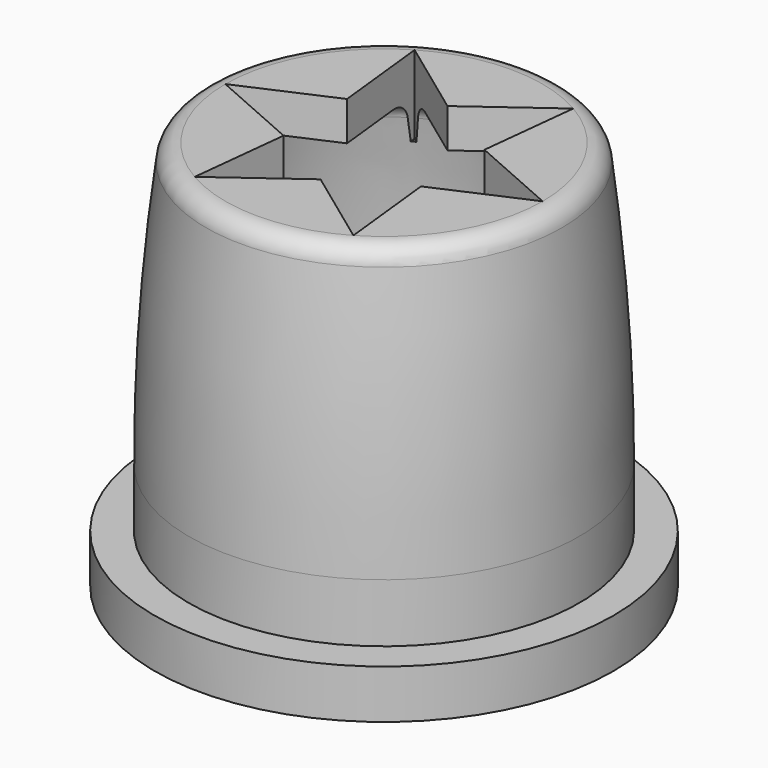
from build123d import *

# Parameters (mm, degrees)
F3_DEPTH    = 4
F4_S6_R     = 8.85
F4_T7_DEPTH = 16


# Not quite as in the source:
# - a fillet or chamfer that OpenCascade refuses, or shapes differently, is made with other operations: its cross-section is extruded or revolved along the edge and cut away or added


with BuildPart() as f1:
    # F0 (on Front) → F1 (revolve)
    with BuildSketch(Plane.XZ):
        with BuildLine():
            Line((-11.75, 2.5), (-11.75, 0))
            Line((-11.75, 0), (-10.45, 0))
            Line((-10.45, 0), (-10.45, 1.2))
            Line((-10.45, 1.2), (-8.85, 1.2))
            Line((-8.85, 1.2), (-8.85, 4.2))
            ThreePointArc((-8.85, 4.2), (-8.5510140246, 10.7185269337), (-7.6565668329, 17.1823145401))
            ThreePointArc((-7.6565668329, 17.1823145401), (-7.3127346822, 17.7688675244), (-6.6733265732, 18))
            Line((-6.6733265732, 18), (0, 18))
            Line((0, 18), (0, 20))
            Line((0, 20), (-8.1253765053, 20))
            ThreePointArc((-8.1253765053, 20), (-8.7852885229, 19.7513428838), (-9.117016902, 19.1290322581))
            ThreePointArc((-9.117016902, 19.1290322581), (-9.7790230738, 12.3288025935), (-10, 5.5))
            Line((-10, 5.5), (-10, 2.5))
            Line((-10, 2.5), (-11.75, 2.5))
        make_face()
    revolve(axis=Axis((0, 0, 19), (0, 0, -1)))

    # F2 (on face) → F3 (cut)
    with BuildSketch(Plane.XY.offset(20)):
        Polygon((4.0626882527, 7.0367824689), (0, 4.0626882527), (-4.0626882527, 7.0367824689), (-3.5183912345, 2.0313441263), (-8.1253765053, 0), (-3.5183912345, -2.0313441263), (-4.0626882527, -7.0367824689), (0, -4.0626882527), (4.0626882527, -7.0367824689), (3.5183912345, -2.0313441263), (8.1253765053, 0), (3.5183912345, 2.0313441263), align=None)
    extrude(amount=-F3_DEPTH, mode=Mode.SUBTRACT)

    # F4: chamfer of 2 on 1 edges, made by hand


with BuildPart() as f4_tool2:
    # F4_s3 → F4_t4 (revolve)
    with BuildSketch(Plane.XZ):
        Polygon((-10.45, -0.8), (-8.45, 1.2), (-10.45, 1.2), align=None)
    revolve(axis=Axis((0, 0, 1.2), (0, 0, -1)))

    split(bisect_by=Plane.XY, keep=Keep.TOP)

    # F4_s6 → F4_t7 (cut, symmetric)
    with BuildSketch(Plane.XY.offset(0.2)):
        Circle(F4_S6_R)
    extrude(amount=F4_T7_DEPTH, both=True, mode=Mode.SUBTRACT)


with BuildPart() as f1_1:
    add(f1.part)

    # F4_t1: union F4_tool2
    add(f4_tool2.part)


solid = f1_1.part
